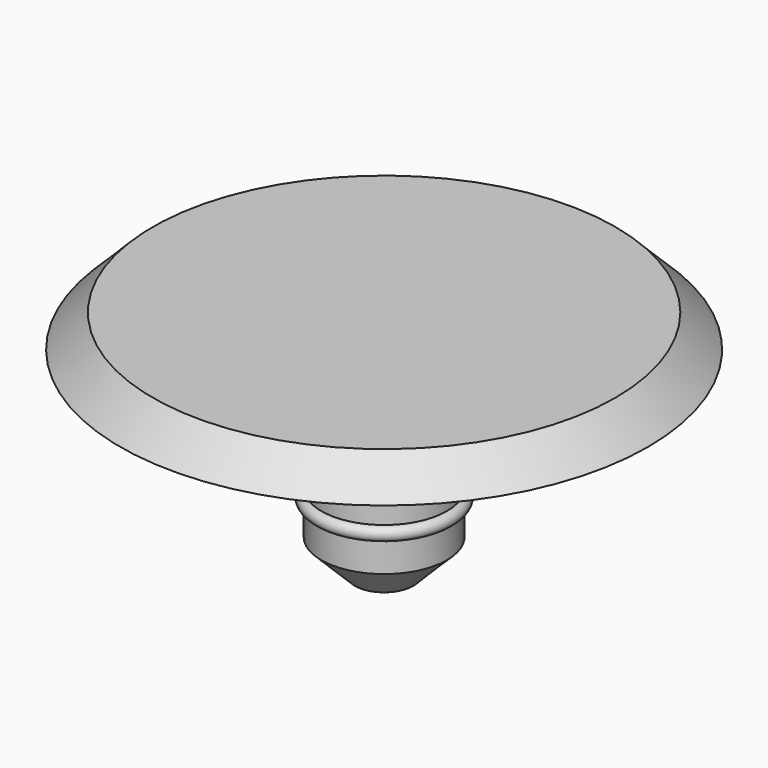
from build123d import *

# Parameters (mm, degrees)
F2_SIZE  = 1.27
F3_R     = 14.2800405429
F3_R_2   = 10
F3_R_3   = 5.842
F4_DEPTH = 0.8
F5_SIZE  = 1.016


# Not quite as in the source:
# - a fillet or chamfer that OpenCascade refuses, or shapes differently, is made with other operations: its cross-section is extruded or revolved along the edge and cut away or added


with BuildPart() as f1:
    # F0 (on Front) → F1 (revolve)
    with BuildSketch(Plane.XZ):
        with BuildLine():
            Line((2.6757909362, 0), (4.2185683136, 0))
            Line((4.2185683136, 0), (10, 0))
            Line((10, 0), (10, 2.032))
            Line((10, 2.032), (0, 2.032))
            Line((0, 2.032), (0, 0))
            Line((0, 0), (0, -6.7))
            Line((0, -6.7), (2.3710267587, -6.7))
            Line((2.3710267587, -6.7), (2.3710267587, -4.308))
            ThreePointArc((2.3710267587, -4.308), (2.6250267587, -4.054), (2.3710267587, -3.8))
            Line((2.3710267587, -3.8), (2.3710267587, 0))
            Line((2.3710267587, 0), (2.6757909362, 0))
        make_face()
    revolve(axis=Axis((0, 0, 1.016), (0, 0, -1)))

    # F2
    f2_edges = [f1.edges().sort_by_distance(p)[0] for p in [
        (-2.371027, 0, -6.7),
    ]]
    chamfer(f2_edges, length=F2_SIZE)

    # F3 (on face) → F4 (cut)
    with BuildSketch(Plane(origin=(0, 0, 0), x_dir=(1, 0, 0), z_dir=(0, 0, -1))):
        Circle(F3_R)
        Circle(F3_R_2, mode=Mode.SUBTRACT)
        Circle(F3_R_2)
        Circle(F3_R_3, mode=Mode.SUBTRACT)
    extrude(amount=-F4_DEPTH, mode=Mode.SUBTRACT)

    # F5
    f5_edges = [f1.edges().sort_by_distance(p)[0] for p in [
        (-2.371027, 0, 0),
    ]]
    chamfer(f5_edges, length=F5_SIZE)

    # F6: chamfer of 1.27 on 1 edges, made by hand

    # F6_s1 → F6_t2 (revolve, cut)
    with BuildSketch(Plane.XZ):
        Polygon((10, 0.762), (8.73, 2.032), (10, 2.032), align=None)
    revolve(axis=Axis((0, 0, 2.032), (0, 0, -1)), mode=Mode.SUBTRACT)


solid = f1.part
